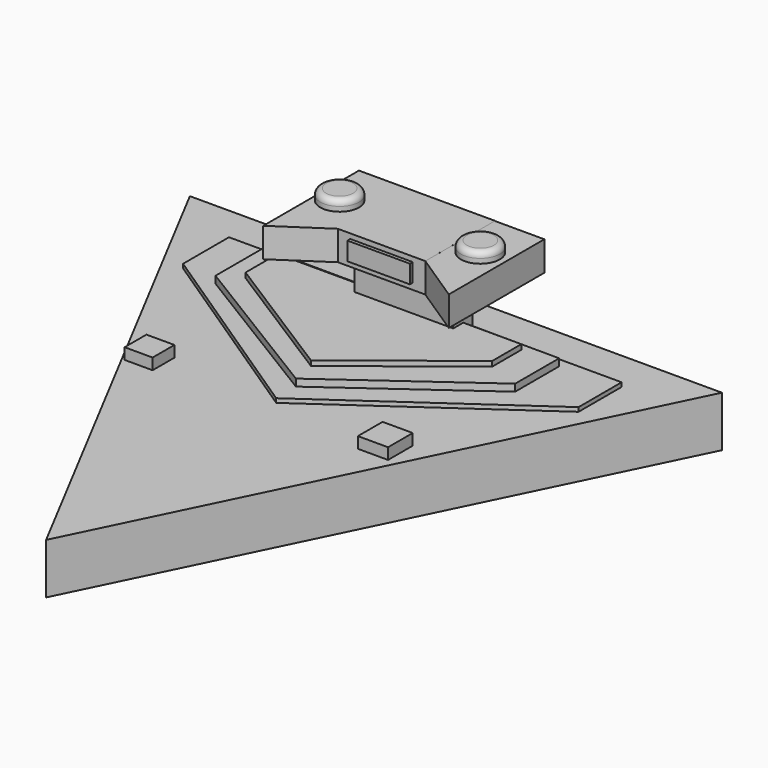
from build123d import *

# Parameters (mm, degrees)
F0_W      = 75.3890946507
F0_H      = 75.1791000366
F1_DEPTH  = 25.4
F4_DEPTH  = 25.4
F5_DEPTH  = 25.4508
F6_W      = 53.92798502
F6_H      = 15.7025610097
F7_DEPTH  = 3.048
F8_W      = 85.17449582
F8_H      = 20.9367480129
F9_DEPTH  = 50.038
F11_DEPTH = 43.688
F12_R     = 17.2027842211
F13_DEPTH = 6.096
F12_R_2   = 17.4931921262
F12_R_3   = 16.7744326075
F15_DEPTH = 3.556
F17_DEPTH = 6.096
F18_W     = 24.1459421813
F18_H     = 23.5268175602
F18_W_2   = 26.0033160448
F18_H_2   = 26.6224443913
F19_DEPTH = 9.652
F20_W     = 56.3405365683
F20_H     = 140.5417844653
F21_DEPTH = 2.54
F23_DEPTH = 4.318
F24_R     = 16.7164206505
F25_DEPTH = 9.144
F24_R_2   = 16.7622193937
F26_R     = 5.08
F26_2_R   = 5.08
F27_R     = 50.773582489
F28_DEPTH = 25.4


# Not quite as in the source:
# - a fillet or chamfer that OpenCascade refuses, or shapes differently, is made with other operations: its cross-section is extruded or revolved along the edge and cut away or added


with BuildPart() as f1:
    # F0 (on Top) → F1 (new body)
    with BuildSketch(Plane.XY):
        with Locations((37.6945473254, -37.5895500183)):
            Rectangle(F0_W, F0_H)
    extrude(amount=F1_DEPTH)

    # F2 (on face) → F4 (join)
    with BuildSketch(Plane.XY.offset(25.4)):
        Polygon((0, -75.1791000366), (0, 0), (-42.0155413449, 0), (-42.0155413449, -103.1650602818), align=None)
    extrude(amount=-F4_DEPTH)


with BuildPart() as f5:
    # F3 (on face) → F5 (new body)
    with BuildSketch(Plane.XY.offset(25.4)):
        Polygon((118.1067675352, -0.2493217471), (75.7626965642, -0.2493217471), (75.3957405686, -0.2493217471), (75.3957405686, -75.1837566495), (118.1067675352, -103.2613441348), align=None)
    extrude(amount=-F5_DEPTH)


with BuildPart() as f7:
    # F6 (on face) → F7 (new body)
    with BuildSketch(Plane.XZ.offset(75.1791000366)):
        with Locations((37.5697775744, 13.2790950593)):
            Rectangle(F6_W, F6_H)
    extrude(amount=F7_DEPTH)


with BuildPart() as f9:
    # F8 (on face) → F9 (new body)
    with BuildSketch(Plane(origin=(0, 0, 0), x_dir=(1, 0, 0), z_dir=(0, 0, -1))):
        with Locations((35.1112957578, 37.4959344044)):
            Rectangle(F8_W, F8_H)
    extrude(amount=F9_DEPTH)

    # F10 (on face) → F11 (join)
    with BuildSketch(Plane(origin=(0, 0, -50.038), x_dir=(1, 0, 0), z_dir=(0, 0, -1))):
        Polygon((260.7715725899, -12.8838187084), (39.4802503288, 439.1739666462), (-198.1444954872, -12.8838187084), align=None)
    extrude(amount=F11_DEPTH)

    # F14 (on face) → F15 (join)
    with BuildSketch(Plane(origin=(0, 0, -50.038), x_dir=(1, 0, 0), z_dir=(0, 0, -1))):
        Polygon((-135.8506828547, 72.3413750529), (-135.8506828547, 31.4790122211), (-135.8506828547, 22.8112302721), (202.8116434813, 22.8112302721), (202.8116434813, 69.2457407713), (35.6474258006, 186.2607002258), align=None)
    extrude(amount=-F15_DEPTH)

    # F16 (on face) → F17 (join)
    with BuildSketch(Plane.XY.offset(-46.482)):
        Polygon((-7.4759521522, -30.1380986139), (-100.561901927, -29.6938885003), (-100.561901927, -81.4376845956), (35.4353301227, -164.7797524929), (155.4093956947, -78.3358365297), (155.4093956947, -30.9153944254), (77.6985436678, -30.5445549325), (77.6985436678, -47.9643084109), (-7.4759521522, -47.9643084109), align=None)
    extrude(amount=F17_DEPTH)

    # F18 (on face) → F19 (join)
    with BuildSketch(Plane.XY.offset(-50.038)):
        with Locations((-71.1519364268, -189.3563270569)):
            Rectangle(F18_W, F18_H)
        with Locations((133.4694549441, -190.9041404724)):
            Rectangle(F18_W_2, F18_H_2)
    extrude(amount=F19_DEPTH)

    # F22 (on face) → F23 (join)
    with BuildSketch(Plane.XY.offset(-40.386)):
        Polygon((127.8130114079, -37.2119806707), (-82.5328603387, -37.0825752616), (-82.5328603387, -71.5653449297), (31.8256095052, -144.0929919481), (127.8130114079, -68.7100365758), align=None)
    extrude(amount=F23_DEPTH)

    # F27 (on face) → F28 (join)
    with BuildSketch(Plane(origin=(0, 0, -93.726), x_dir=(1, 0, 0), z_dir=(0, 0, -1))):
        with Locations((31.8289473653, 62.0807632804)):
            Circle(F27_R)
    extrude(amount=F28_DEPTH)

    # F29: fillet of radius 42.924717139 on 1 edges, made by hand

    # F29_s1 → F29_t2 (revolve, cut)
    with BuildSketch(Plane.XZ.offset(62.0807632804)):
        with BuildLine():
            ThreePointArc((82.6025298543, -93.726), (66.7664669422, -112.2205476203), (43.4181499222, -119.126))
            Line((43.4181499222, -119.126), (82.6025298543, -119.126))
            Line((82.6025298543, -119.126), (82.6025298543, -93.726))
        make_face()
    revolve(axis=Axis((31.8289473653, -62.0807632804, -119.126), (0, 0, -1)), mode=Mode.SUBTRACT)


with BuildPart() as f13:
    # F12 (on face) → F13 (new body)
    with BuildSketch(Plane(origin=(0, 12.8838187084, 0), x_dir=(-1, 0, 0), z_dir=(0, 1, 0))):
        with Locations((-38.6442020535, -71.5526640415)):
            Circle(F12_R)
    extrude(amount=F13_DEPTH)


with BuildPart() as f13b:
    # F12 (on face) → F13, piece 2 (new body)
    with BuildSketch(Plane(origin=(0, 12.8838187084, 0), x_dir=(-1, 0, 0), z_dir=(0, 1, 0))):
        with Locations((-180.981323123, -71.5526640415)):
            Circle(F12_R_2)
    extrude(amount=F13_DEPTH)


with BuildPart() as f13c:
    # F12 (on face) → F13, piece 3 (new body)
    with BuildSketch(Plane(origin=(0, 12.8838187084, 0), x_dir=(-1, 0, 0), z_dir=(0, 1, 0))):
        with Locations((118.9651414752, -71.5526640415)):
            Circle(F12_R_3)
    extrude(amount=F13_DEPTH)


with BuildPart() as f21:
    # F20 (on face) → F21 (new body)
    with BuildSketch(Plane(origin=(0, 0, -93.726), x_dir=(1, 0, 0), z_dir=(0, 0, -1))):
        with Locations((35.9569906723, 193.3806575835)):
            Rectangle(F20_W, F20_H)
    extrude(amount=F21_DEPTH)


with BuildPart() as f25:
    # F24 (on face) → F25 (new body)
    with BuildSketch(Plane.XY.offset(25.4)):
        with Locations((-25.0269956887, -42.0041643083)):
            Circle(F24_R)
    extrude(amount=F25_DEPTH)

    # F26
    f26_edges = [f25.edges().sort_by_distance(p)[0] for p in [
        (-41.743416, -42.004164, 34.544),
    ]]
    fillet(f26_edges, radius=F26_R)


with BuildPart() as f25b:
    # F24 (on face) → F25, piece 2 (new body)
    with BuildSketch(Plane.XY.offset(25.4)):
        with Locations((96.3218435645, -42.0041643083)):
            Circle(F24_R_2)
    extrude(amount=F25_DEPTH)

    # F26#2
    f26_2_edges = [f25b.edges().sort_by_distance(p)[0] for p in [
        (79.559624, -42.004164, 34.544),
    ]]
    fillet(f26_2_edges, radius=F26_2_R)


solid = Compound([f1.part, f5.part, f7.part, f9.part, f13.part, f13b.part, f13c.part, f21.part, f25.part, f25b.part])
